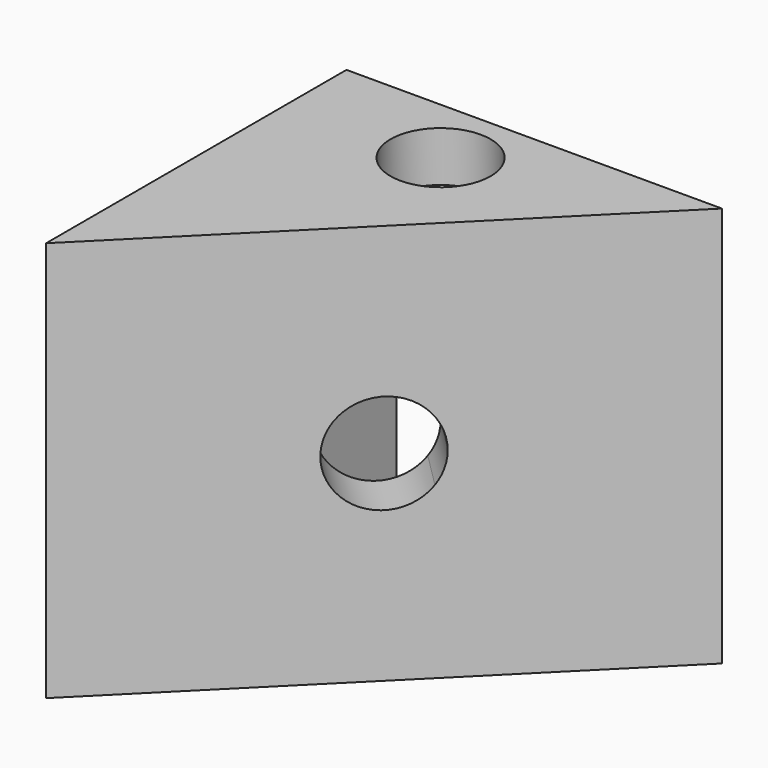
from build123d import *

# Parameters (mm, degrees)
F1_DEPTH = 25.4
F2_T     = -3.175
F3_DEPTH = 25.4
F4_R     = 3.175
F5_DEPTH = 3.175
F6_R     = 3.175
F7_DEPTH = 25.4
F9_DEPTH = 3.175


# Not quite as in the source:
# - a feature names something its author has since deleted; it is built from what else it names


with BuildPart() as f1:
    # F0 (on Top) → F1 (new body)
    with BuildSketch(Plane.XY):
        Polygon((11.90625, 11.90625), (-11.90625, 11.90625), (-11.90625, -11.90625), align=None)
    extrude(amount=F1_DEPTH)

    # F2
    f2_openings = [f1.faces().sort_by_distance(p)[0] for p in [
        (0, 11.90625, 12.7),
    ]]
    offset(amount=F2_T, openings=f2_openings)

    # F3 (cut): a face of the model
    f3_faces = [f1.faces().sort_by_distance(p)[0] for p in [
        (-3.3487926868, 6.5237926868, 3.175),
    ]]
    extrude(f3_faces, amount=-F3_DEPTH, mode=Mode.SUBTRACT)

    # F4 (on face) → F5 (cut)
    with BuildSketch(Plane(origin=(-11.90625, 0, 0), x_dir=(0, -1, 0), z_dir=(-1, 0, 0))):
        with Locations((-2.38125, 12.7)):
            Circle(F4_R)
    extrude(amount=-F5_DEPTH, mode=Mode.SUBTRACT)

    # F6 (on face) → F7 (cut)
    with BuildSketch(Plane.XY.offset(25.4)):
        with Locations((-2.38125, 7.46125)):
            Circle(F6_R)
    extrude(amount=-F7_DEPTH, mode=Mode.SUBTRACT)

    # F8 (on face) → F9 (cut)
    with BuildSketch(Plane(origin=(0, 0, 0), x_dir=(0.7071067812, 0.7071067812, 0), z_dir=(0.7071067812, -0.7071067812, 0))):
        with BuildLine():
            ThreePointArc((3.175, 12.7), (1.0081076412, 15.7107048982), (-2.5348229819, 14.6118832209))
            Line((-2.5348229819, 14.6118832209), (2.5348229819, 10.7881167791))
            ThreePointArc((2.5348229819, 10.7881167791), (3.0107048982, 11.6918923588), (3.175, 12.7))
        make_face()
        with BuildLine():
            Line((2.5348229819, 10.7881167791), (-2.5348229819, 14.6118832209))
            ThreePointArc((-2.5348229819, 14.6118832209), (-1.9118832209, 10.1651770181), (2.5348229819, 10.7881167791))
        make_face()
    extrude(amount=-F9_DEPTH, mode=Mode.SUBTRACT)


solid = f1.part
